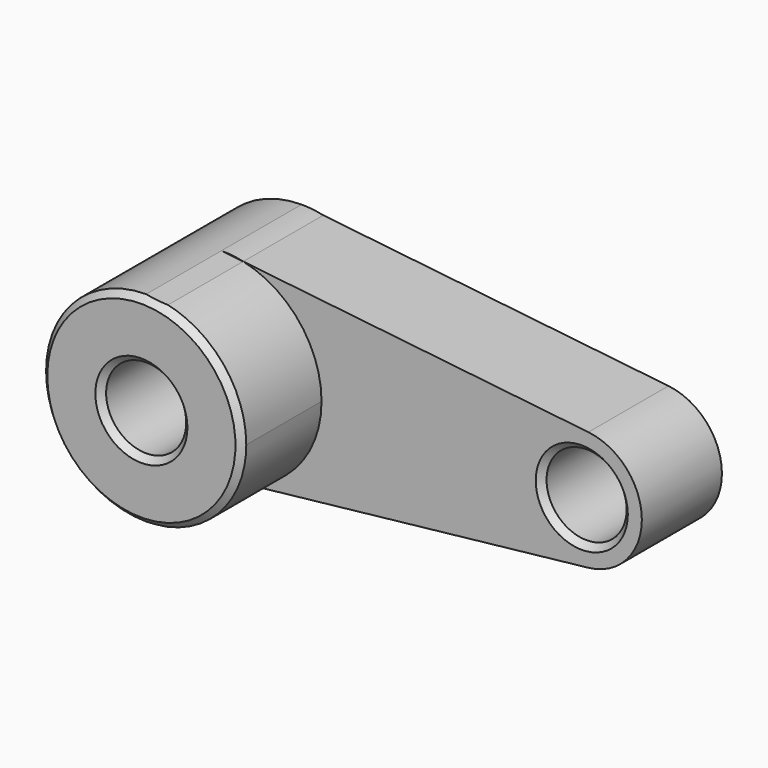
from build123d import *

# Parameters (mm, degrees)
F0_R        = 10
F1_DEPTH    = 25
F2_DEPTH    = 50
F3_T4_ANGLE = 197.7100251144
F3_T6_ANGLE = 172.569908128


# Not quite as in the source:
# - a fillet or chamfer that OpenCascade refuses, or shapes differently, is made with other operations: its cross-section is extruded or revolved along the edge and cut away or added


with BuildPart() as f1:
    # F0 (on Front) → F1 (new body)
    with BuildSketch(Plane.XZ):
        with BuildLine():
            Line((5.4392563459, 24.4011165811), (0, 25))
            ThreePointArc((0, 25), (-25, 0), (0, -25))
            Line((0, -25), (5.4392563459, -24.4011165811))
            ThreePointArc((5.4392563459, -24.4011165811), (19.5061709293, -15.6367930113), (25, 0))
            ThreePointArc((25, 0), (19.5061709293, 15.6367930113), (5.4392563459, 24.4011165811))
        make_face()
        Circle(F0_R, mode=Mode.SUBTRACT)
        with BuildLine():
            ThreePointArc((5.4392563459, 24.4011165811), (2.7360633648, 24.8498281134), (0, 25))
            Line((0, 25), (5.4392563459, 24.4011165811))
        make_face()
        with BuildLine():
            Line((5.4392563459, -24.4011165811), (0, -25))
            ThreePointArc((0, -25), (2.7360633648, -24.8498281134), (5.4392563459, -24.4011165811))
        make_face()
        with BuildLine():
            Line((91.6416380189, 14.909896868), (5.4392563459, 24.4011165811))
            ThreePointArc((5.4392563459, 24.4011165811), (19.5061709293, 15.6367930113), (25, 0))
            ThreePointArc((25, 0), (19.5061709293, -15.6367930113), (5.4392563459, -24.4011165811))
            Line((5.4392563459, -24.4011165811), (91.6416380189, -14.909896868))
            ThreePointArc((91.6416380189, -14.909896868), (75, 0), (91.6416380189, 14.909896868))
        make_face()
        with BuildLine():
            ThreePointArc((105, 0), (101.1719418698, 10.0093813424), (91.6416380189, 14.909896868))
            ThreePointArc((91.6416380189, 14.909896868), (75, 0), (91.6416380189, -14.909896868))
            ThreePointArc((91.6416380189, -14.909896868), (101.1719418698, -10.0093813424), (105, 0))
        make_face()
        with Locations((90, 0)):
            Circle(F0_R, mode=Mode.SUBTRACT)
    extrude(amount=F1_DEPTH)

    # F0 (on Front) → F2 (join)
    with BuildSketch(Plane.XZ):
        with BuildLine():
            Line((5.4392563459, 24.4011165811), (0, 25))
            ThreePointArc((0, 25), (-25, 0), (0, -25))
            Line((0, -25), (5.4392563459, -24.4011165811))
            ThreePointArc((5.4392563459, -24.4011165811), (19.5061709293, -15.6367930113), (25, 0))
            ThreePointArc((25, 0), (19.5061709293, 15.6367930113), (5.4392563459, 24.4011165811))
        make_face()
        Circle(F0_R, mode=Mode.SUBTRACT)
    extrude(amount=F2_DEPTH)

    # F3: chamfer of 1.5 on 4 edges, made by hand

    # F3_s1 → F3_t2 (revolve, cut)
    with BuildSketch(Plane.XY):
        with BuildLine():
            Line((11.5424264069, -50.0424264069), (9.9575735931, -48.4575735931))
            Line((9.9575735931, -48.4575735931), (9.9275735931, -48.4575735931))
            ThreePointArc((9.9275735931, -48.4575735931), (9.97, -49.2287867966), (9.97, -50))
            Line((9.97, -50), (10, -50.03))
            ThreePointArc((10, -50.03), (10.7712132034, -50.03), (11.5424264069, -50.0724264069))
            Line((11.5424264069, -50.0724264069), (11.5424264069, -50.0424264069))
        make_face()
    revolve(axis=Axis((0, -50, 0), (0, -1, 0)), mode=Mode.SUBTRACT)

    # F3_s3 → F3_t4 (revolve, cut)
    with BuildSketch(Plane(origin=(0, 0, 0), x_dir=(0, 1, 0), z_dir=(0.9880810366, 0, -0.1539346134))):
        with BuildLine():
            Line((-48.4575735931, 25.0424264069), (-50.0424264069, 23.4575735931))
            Line((-50.0424264069, 23.4575735931), (-50.0724264069, 23.4575735931))
            ThreePointArc((-50.0724264069, 23.4575735931), (-50.03, 24.2287867966), (-50.03, 25))
            Line((-50.03, 25), (-50, 25.03))
            ThreePointArc((-50, 25.03), (-49.2287867966, 25.03), (-48.4575735931, 25.0724264069))
            Line((-48.4575735931, 25.0724264069), (-48.4575735931, 25.0424264069))
        make_face()
    revolve(axis=Axis((0, -50, 0), (0, -1, 0)), revolution_arc=F3_T4_ANGLE, mode=Mode.SUBTRACT)

    # F3_s5 → F3_t6 (revolve, cut)
    with BuildSketch(Plane(origin=(0, 0, 0), x_dir=(0, 1, 0), z_dir=(-0.9978986376, 0, 0.0647943598))):
        with BuildLine():
            Line((-48.4575735931, -25.0424264069), (-50.0424264069, -23.4575735931))
            Line((-50.0424264069, -23.4575735931), (-50.0724264069, -23.4575735931))
            ThreePointArc((-50.0724264069, -23.4575735931), (-50.03, -24.2287867966), (-50.03, -25))
            Line((-50.03, -25), (-50, -25.03))
            ThreePointArc((-50, -25.03), (-49.2287867966, -25.03), (-48.4575735931, -25.0724264069))
            Line((-48.4575735931, -25.0724264069), (-48.4575735931, -25.0424264069))
        make_face()
    revolve(axis=Axis((0, -50, 0), (0, 1, 0)), revolution_arc=F3_T6_ANGLE, mode=Mode.SUBTRACT)

    # F3_s7 → F3_t8 (revolve, cut)
    with BuildSketch(Plane.XY):
        with BuildLine():
            Line((101.5424264069, -25.0424264069), (99.9575735931, -23.4575735931))
            Line((99.9575735931, -23.4575735931), (99.9275735931, -23.4575735931))
            ThreePointArc((99.9275735931, -23.4575735931), (99.97, -24.2287867966), (99.97, -25))
            Line((99.97, -25), (100, -25.03))
            ThreePointArc((100, -25.03), (100.7712132034, -25.03), (101.5424264069, -25.0724264069))
            Line((101.5424264069, -25.0724264069), (101.5424264069, -25.0424264069))
        make_face()
    revolve(axis=Axis((90, -25, 0), (0, -1, 0)), mode=Mode.SUBTRACT)


solid = f1.part
